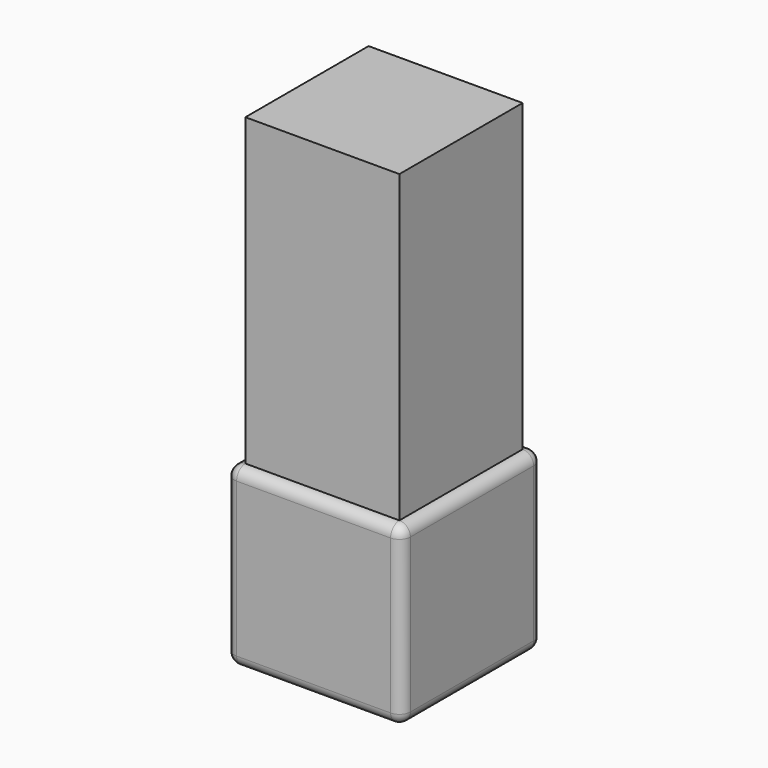
from build123d import *

# Parameters (mm, degrees)
F0_W     = 80
F0_H     = 80
F1_DEPTH = 40
F2_R     = 5
F3_DEPTH = 80.001


# Not quite as in the source:
# - a pattern or mirror of a feature is missing from the dataset's text; its kind, count and spacing are read off the source's solid


with BuildPart() as f1:
    # F0 (on Top) → F1 (new body, symmetric)
    with BuildSketch(Plane.XY):
        Rectangle(F0_W, F0_H)
    extrude(amount=F1_DEPTH, both=True)

    # F2
    f2_edges = [f1.edges().sort_by_distance(p)[0] for p in [
        (0, 40, 40),
        (-40, 0, 40),
        (40, 0, 40),
        (0, -40, 40),
        (40, 40, 0),
        (40, -40, 0),
        (40, 0, -40),
        (-40, 40, 0),
        (-40, 0, -40),
        (-40, -40, 0),
        (0, -40, -40),
        (0, 40, -40),
    ]]
    fillet(f2_edges, radius=F2_R)

    # F3 (add, through all): faces of the model
    f3_faces = [f1.faces().sort_by_distance(p)[0] for p in [
        (0, 0, -40),
        (0, 0, 40),
    ]]
    f3 = extrude(f3_faces, amount=-F3_DEPTH, dir=(0, 0, -1))

    # F3_copies: F3 across plane
    add(f3.mirror(Plane.XY.offset(69.287032)))


solid = f1.part
